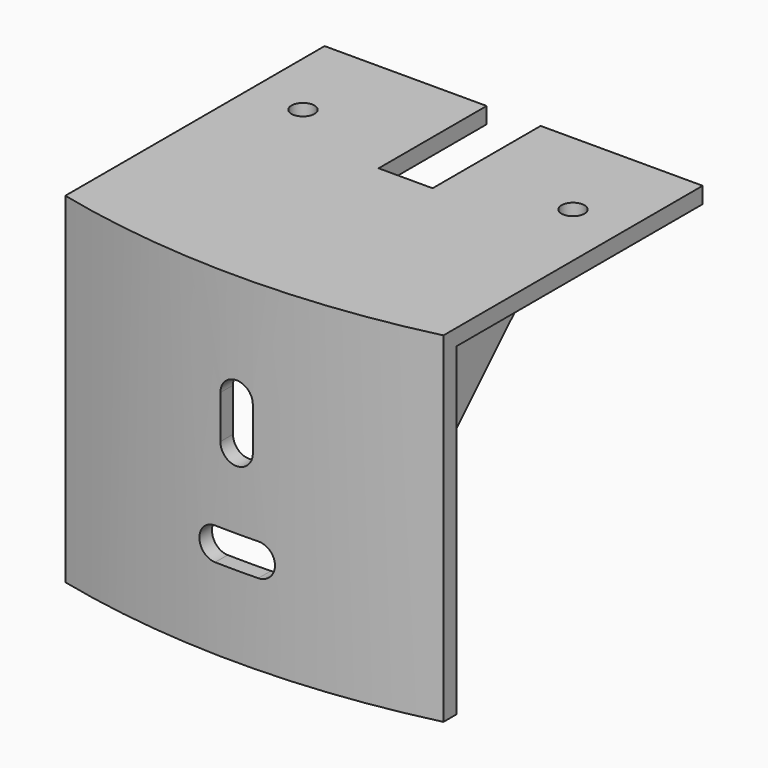
from build123d import *

# Parameters (mm, degrees)
F0_R     = 4.25
F1_DEPTH = 6
F3_DEPTH = 120
F5_DEPTH = 120
F7_REACH = 132.1169232427
F9_DEPTH = 300.001


with BuildPart() as f1:
    # F0 (on Top) → F1 (new body)
    with BuildSketch(Plane.XY):
        with BuildLine():
            Line((-70, -171.7190429163), (-70, -291.7190429163))
            ThreePointArc((-70, -291.7190429163), (0, -300), (70, -291.7190429163))
            Line((70, -291.7190429163), (70, -171.7190429163))
            Line((70, -171.7190429163), (10, -171.7190429163))
            Line((10, -171.7190429163), (10, -221.7190429163))
            Line((10, -221.7190429163), (0, -221.7190429163))
            Line((0, -221.7190429163), (-10, -221.7190429163))
            Line((-10, -221.7190429163), (-10, -171.7190429163))
            Line((-10, -171.7190429163), (-70, -171.7190429163))
        make_face()
        with Locations((-50, -206.7190429163)):
            Circle(F0_R, mode=Mode.SUBTRACT)
        with Locations((50, -206.7190429163)):
            Circle(F0_R, mode=Mode.SUBTRACT)
    extrude(amount=-F1_DEPTH)

    # F2 (on face) → F3 (join)
    with BuildSketch(Plane(origin=(0, 0, -6), x_dir=(1, 0, 0), z_dir=(0, 0, -1))):
        with BuildLine():
            Line((-54, 237.9850195496), (-54, 289.1701427966))
            ThreePointArc((-54, 289.1701427966), (-57.0030799982, 288.5931744788), (-60, 287.9850195496))
            Line((-60, 287.9850195496), (-60, 237.9850195496))
            Line((-60, 237.9850195496), (-54, 237.9850195496))
        make_face()
        with BuildLine():
            ThreePointArc((60, 287.9850195496), (65.0098735772, 286.8956043973), (70, 285.7190429163))
            Line((70, 285.7190429163), (70, 291.7190429163))
            ThreePointArc((70, 291.7190429163), (0, 300), (-70, 291.7190429163))
            Line((-70, 291.7190429163), (-70, 285.7190429163))
            ThreePointArc((-70, 285.7190429163), (-65.0098735772, 286.8956043973), (-60, 287.9850195496))
            ThreePointArc((-60, 287.9850195496), (-57.0030799982, 288.5931744788), (-54, 289.1701427966))
            ThreePointArc((-54, 289.1701427966), (0, 294.1689505794), (54, 289.1701427966))
            ThreePointArc((54, 289.1701427966), (57.0030799982, 288.5931744788), (60, 287.9850195496))
        make_face()
        with BuildLine():
            Line((60, 237.9850195496), (60, 287.9850195496))
            ThreePointArc((60, 287.9850195496), (57.0030799982, 288.5931744788), (54, 289.1701427966))
            Line((54, 289.1701427966), (54, 237.9850195496))
            Line((54, 237.9850195496), (60, 237.9850195496))
        make_face()
    extrude(amount=F3_DEPTH)

    # F4 (on face) → F5 (cut, through all)
    with BuildSketch(Plane.YZ.offset(60)):
        Polygon((-237.9850195496, -126), (-237.9850195496, -6), (-287.9850195496, -56), (-287.9850195496, -126), align=None)
    extrude(amount=-F5_DEPTH, mode=Mode.SUBTRACT)

    f7_end = Plane(origin=(57, -262.9850195496, -31), x_dir=(0, 0.7071067812, 0.7071067812), z_dir=(0, 0.7071067812, -0.7071067812))
    # F6 (on face) → F7 (cut, up to a plane its end follows)
    with BuildSketch(Plane(origin=(0, 0, -126), x_dir=(1, 0, 0), z_dir=(0, 0, -1))):
        Polygon((-54, 287.9850195496), (-54, 289.1701427966), (-60, 287.9850195496), align=None)
        Polygon((60, 287.9850195496), (54, 289.1701427966), (54, 287.9850195496), align=None)
    f7_long = extrude(amount=-F7_REACH, mode=Mode.PRIVATE)
    add(split(f7_long, bisect_by=f7_end, keep=Keep.TOP, mode=Mode.PRIVATE), mode=Mode.SUBTRACT)

    # F8 (on Front) → F9 (cut, through all)
    with BuildSketch(Plane.XZ):
        with BuildLine():
            Line((8, -84), (0, -84))
            Line((0, -84), (-8, -84))
            ThreePointArc((-8, -84), (-14, -90), (-8, -96))
            Line((-8, -96), (0, -96))
            Line((0, -96), (8, -96))
            ThreePointArc((8, -96), (14, -90), (8, -84))
        make_face()
        with BuildLine():
            Line((6, -48), (6, -40))
            ThreePointArc((6, -40), (0, -34), (-6, -40))
            Line((-6, -40), (-6, -48))
            Line((-6, -48), (-6, -56))
            ThreePointArc((-6, -56), (0, -62), (6, -56))
            Line((6, -56), (6, -48))
        make_face()
    extrude(amount=F9_DEPTH, mode=Mode.SUBTRACT)


solid = f1.part
